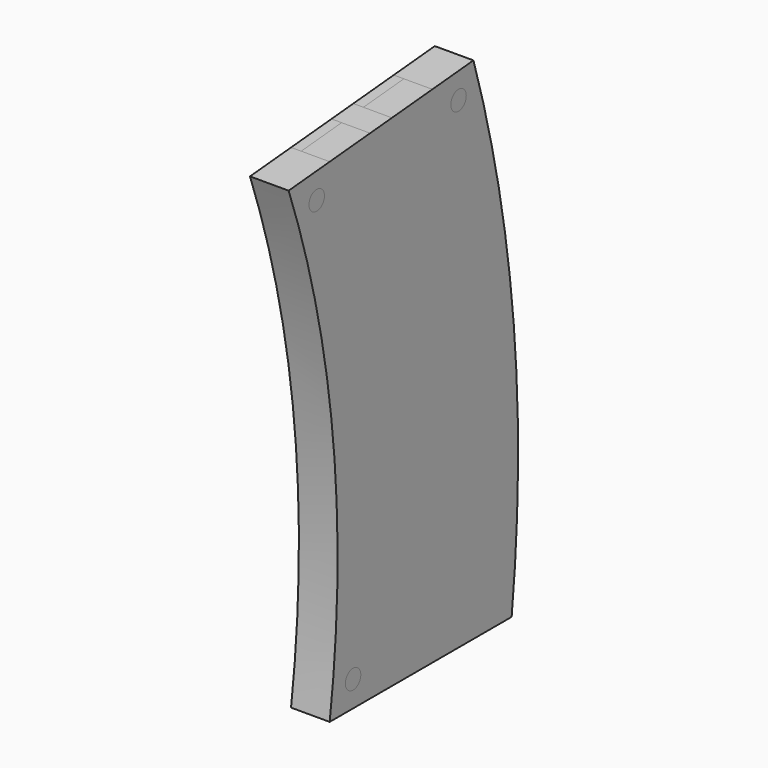
from build123d import *

# Parameters (mm, degrees)
F0_R     = 4.7625
F1_DEPTH = 19.05
F2_DEPTH = 8
F3_DEPTH = 19.05
F4_DEPTH = 8
F5_DEPTH = 19.05
F6_DEPTH = 5


with BuildPart() as f1:
    # F0 (on Right) → F1 (new body)
    with BuildSketch(Plane.YZ):
        with BuildLine():
            Line((72.1463597932, 149.9590638802), (85.6583556438, 0))
            Line((85.6583556438, 0), (112.083494131, 0))
            ThreePointArc((112.083494131, 0), (113.3609778359, 126.7442629535), (88.5413006025, 251.0411807683))
            Line((88.5413006025, 251.0411807683), (63.2437861446, 248.7617592946))
            Line((63.2437861446, 248.7617592946), (72.1463597932, 149.9590638802))
        make_face()
        with Locations((79.3634283737, 237.4627622397)):
            Circle(F0_R, mode=Mode.SUBTRACT)
        Polygon((8.9025736486, 144.260510196), (21.9011038124, 0), (85.6583556438, 0), (72.1463597932, 149.9590638802), (47.2472313898, 147.7155388077), (33.801702052, 146.5040352685), align=None)
        Polygon((0, 243.0632056103), (8.9025736486, 144.260510196), (33.801702052, 146.5040352685), (24.8991284034, 245.3067306829), align=None)
        Polygon((47.2472313898, 147.7155388077), (72.1463597932, 149.9590638802), (63.2437861446, 248.7617592946), (38.3446577412, 246.518234222), align=None)
        Polygon((24.8991284034, 245.3067306829), (33.801702052, 146.5040352685), (47.2472313898, 147.7155388077), (38.3446577412, 246.518234222), align=None)
        with Locations((79.3634283737, 237.4627622397)):
            Circle(F0_R)
        with BuildLine():
            ThreePointArc((-25.2975144579, 240.7837841366), (2.0929056904, 121.9406983227), (0, 0))
            Line((0, 0), (21.9011038124, 0))
            Line((21.9011038124, 0), (8.9025736486, 144.260510196))
            Line((8.9025736486, 144.260510196), (0, 243.0632056103))
            Line((0, 243.0632056103), (-25.2975144579, 240.7837841366))
        make_face()
        with Locations((14.3920474864, 12.7)):
            Circle(F0_R, mode=Mode.SUBTRACT)
        with Locations((-8.0000355449, 229.5909155409)):
            Circle(F0_R, mode=Mode.SUBTRACT)
        with Locations((14.3920474864, 12.7)):
            Circle(F0_R)
        with Locations((-8.0000355449, 229.5909155409)):
            Circle(F0_R)
    extrude(amount=F1_DEPTH)

    # F0 (on Right) → F2 (cut)
    with BuildSketch(Plane.YZ):
        with Locations((79.3634283737, 237.4627622397)):
            Circle(F0_R)
        with Locations((-8.0000355449, 229.5909155409)):
            Circle(F0_R)
        with Locations((14.3920474864, 12.7)):
            Circle(F0_R)
    extrude(amount=F2_DEPTH, mode=Mode.SUBTRACT)


with BuildPart() as f3:
    # F0 (on Right) → F3 (new body)
    with BuildSketch(Plane.YZ):
        with BuildLine():
            Line((72.1463597932, 149.9590638802), (85.6583556438, 0))
            Line((85.6583556438, 0), (112.083494131, 0))
            ThreePointArc((112.083494131, 0), (113.3609778359, 126.7442629535), (88.5413006025, 251.0411807683))
            Line((88.5413006025, 251.0411807683), (63.2437861446, 248.7617592946))
            Line((63.2437861446, 248.7617592946), (72.1463597932, 149.9590638802))
        make_face()
        with Locations((79.3634283737, 237.4627622397)):
            Circle(F0_R, mode=Mode.SUBTRACT)
        Polygon((47.2472313898, 147.7155388077), (72.1463597932, 149.9590638802), (63.2437861446, 248.7617592946), (38.3446577412, 246.518234222), align=None)
        Polygon((24.8991284034, 245.3067306829), (33.801702052, 146.5040352685), (47.2472313898, 147.7155388077), (38.3446577412, 246.518234222), align=None)
        Polygon((0, 243.0632056103), (8.9025736486, 144.260510196), (33.801702052, 146.5040352685), (24.8991284034, 245.3067306829), align=None)
        with BuildLine():
            ThreePointArc((-25.2975144579, 240.7837841366), (2.0929056904, 121.9406983227), (0, 0))
            Line((0, 0), (21.9011038124, 0))
            Line((21.9011038124, 0), (8.9025736486, 144.260510196))
            Line((8.9025736486, 144.260510196), (0, 243.0632056103))
            Line((0, 243.0632056103), (-25.2975144579, 240.7837841366))
        make_face()
        with Locations((14.3920474864, 12.7)):
            Circle(F0_R, mode=Mode.SUBTRACT)
        with Locations((-8.0000355449, 229.5909155409)):
            Circle(F0_R, mode=Mode.SUBTRACT)
        Polygon((8.9025736486, 144.260510196), (21.9011038124, 0), (85.6583556438, 0), (72.1463597932, 149.9590638802), (47.2472313898, 147.7155388077), (33.801702052, 146.5040352685), align=None)
    extrude(amount=F3_DEPTH)

    # F0 (on Right) → F4 (cut)
    with BuildSketch(Plane.YZ):
        Polygon((8.9025736486, 144.260510196), (21.9011038124, 0), (85.6583556438, 0), (72.1463597932, 149.9590638802), (47.2472313898, 147.7155388077), (33.801702052, 146.5040352685), align=None)
        Polygon((47.2472313898, 147.7155388077), (72.1463597932, 149.9590638802), (63.2437861446, 248.7617592946), (38.3446577412, 246.518234222), align=None)
        Polygon((24.8991284034, 245.3067306829), (33.801702052, 146.5040352685), (47.2472313898, 147.7155388077), (38.3446577412, 246.518234222), align=None)
        Polygon((0, 243.0632056103), (8.9025736486, 144.260510196), (33.801702052, 146.5040352685), (24.8991284034, 245.3067306829), align=None)
    extrude(amount=F4_DEPTH, mode=Mode.SUBTRACT)


with BuildPart() as f5:
    # F0 (on Right) → F5 (new body)
    with BuildSketch(Plane.YZ):
        Polygon((8.9025736486, 144.260510196), (21.9011038124, 0), (85.6583556438, 0), (72.1463597932, 149.9590638802), (47.2472313898, 147.7155388077), (33.801702052, 146.5040352685), align=None)
        with BuildLine():
            Line((72.1463597932, 149.9590638802), (85.6583556438, 0))
            Line((85.6583556438, 0), (112.083494131, 0))
            ThreePointArc((112.083494131, 0), (113.3609778359, 126.7442629535), (88.5413006025, 251.0411807683))
            Line((88.5413006025, 251.0411807683), (63.2437861446, 248.7617592946))
            Line((63.2437861446, 248.7617592946), (72.1463597932, 149.9590638802))
        make_face()
        with Locations((79.3634283737, 237.4627622397)):
            Circle(F0_R, mode=Mode.SUBTRACT)
        Polygon((47.2472313898, 147.7155388077), (72.1463597932, 149.9590638802), (63.2437861446, 248.7617592946), (38.3446577412, 246.518234222), align=None)
        Polygon((24.8991284034, 245.3067306829), (33.801702052, 146.5040352685), (47.2472313898, 147.7155388077), (38.3446577412, 246.518234222), align=None)
        Polygon((0, 243.0632056103), (8.9025736486, 144.260510196), (33.801702052, 146.5040352685), (24.8991284034, 245.3067306829), align=None)
        with BuildLine():
            ThreePointArc((-25.2975144579, 240.7837841366), (2.0929056904, 121.9406983227), (0, 0))
            Line((0, 0), (21.9011038124, 0))
            Line((21.9011038124, 0), (8.9025736486, 144.260510196))
            Line((8.9025736486, 144.260510196), (0, 243.0632056103))
            Line((0, 243.0632056103), (-25.2975144579, 240.7837841366))
        make_face()
        with Locations((14.3920474864, 12.7)):
            Circle(F0_R, mode=Mode.SUBTRACT)
        with Locations((-8.0000355449, 229.5909155409)):
            Circle(F0_R, mode=Mode.SUBTRACT)
    extrude(amount=F5_DEPTH)

    # F0 (on Right) → F6 (cut)
    with BuildSketch(Plane.YZ):
        Polygon((47.2472313898, 147.7155388077), (72.1463597932, 149.9590638802), (63.2437861446, 248.7617592946), (38.3446577412, 246.518234222), align=None)
        Polygon((0, 243.0632056103), (8.9025736486, 144.260510196), (33.801702052, 146.5040352685), (24.8991284034, 245.3067306829), align=None)
    extrude(amount=F6_DEPTH, mode=Mode.SUBTRACT)


solid = Compound([f1.part, f3.part, f5.part])
